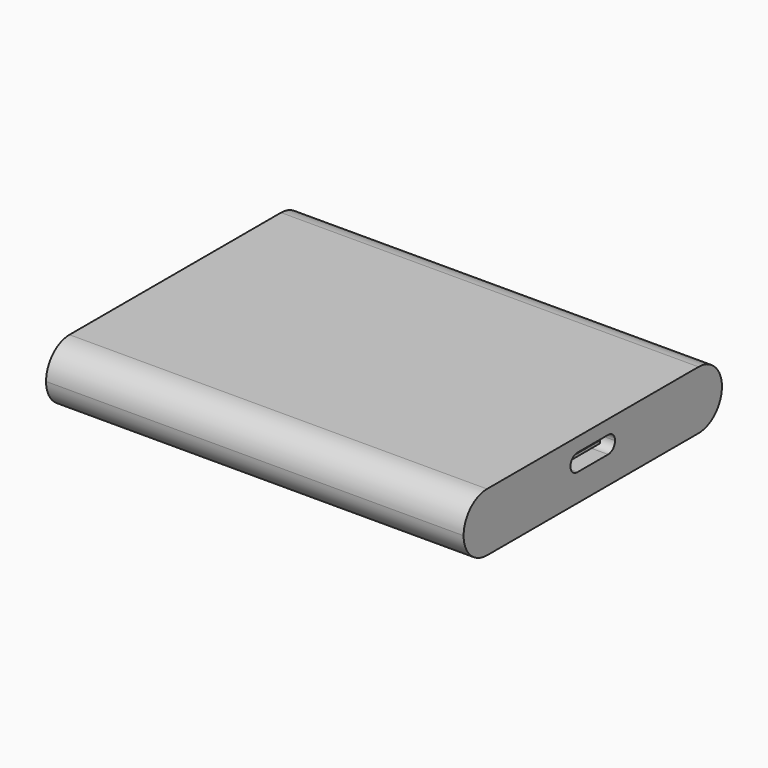
from build123d import *

# Parameters (mm, degrees)
F0_W     = 75
F0_H     = 58
F1_DEPTH = 10.5
F3_R     = 5.24999
F4_DEPTH = 6
F5_W     = 6.9
F5_H     = 0.25
F6_DEPTH = 4.572


# Not quite as in the source:
# - a fillet or chamfer is up to 0.001 mm smaller than in the source, because OpenCascade refuses the exact size


with BuildPart() as f1:
    # F0 (on Top) → F1 (new body)
    with BuildSketch(Plane.XY):
        with Locations((-17.9516240954, -13.4977242947)):
            Rectangle(F0_W, F0_H)
    extrude(amount=F1_DEPTH)

    # F3 (radius 5.25 in the source; OpenCascade refuses exactly that, so slightly less here)
    f3_edges = [f1.edges().sort_by_distance(p)[0] for p in [
        (-17.951624, -42.497724, 10.5),
        (-17.951624, -42.497724, 0),
        (-17.951624, 15.502276, 10.5),
        (-17.951624, 15.502276, 0),
    ]]
    fillet(f3_edges, radius=F3_R)

    # F2 (on face) → F4 (cut)
    with BuildSketch(Plane.YZ.offset(19.5483759046)):
        with BuildLine():
            Line((-10.0477242947, 8), (-13.4977242947, 8))
            Line((-13.4977242947, 8), (-16.9477242947, 8))
            ThreePointArc((-16.9477242947, 8), (-15.8517087838, 7.5460155108), (-15.3977242947, 6.45))
            ThreePointArc((-15.3977242947, 6.45), (-15.8517087838, 5.3539844892), (-16.9477242947, 4.9))
            Line((-16.9477242947, 4.9), (-10.0477242947, 4.9))
            ThreePointArc((-10.0477242947, 4.9), (-11.5977242947, 6.45), (-10.0477242947, 8))
        make_face()
        with BuildLine():
            Line((-10.0477242947, 4.9), (-10.0477242947, 8))
            ThreePointArc((-10.0477242947, 8), (-11.5977242947, 6.45), (-10.0477242947, 4.9))
        make_face()
        with BuildLine():
            ThreePointArc((-8.4977242947, 6.45), (-8.9517087838, 7.5460155108), (-10.0477242947, 8))
            Line((-10.0477242947, 8), (-10.0477242947, 4.9))
            ThreePointArc((-10.0477242947, 4.9), (-8.9517087838, 5.3539844892), (-8.4977242947, 6.45))
        make_face()
        with BuildLine():
            ThreePointArc((-15.3977242947, 6.45), (-15.8517087838, 7.5460155108), (-16.9477242947, 8))
            Line((-16.9477242947, 8), (-16.9477242947, 4.9))
            ThreePointArc((-16.9477242947, 4.9), (-15.8517087838, 5.3539844892), (-15.3977242947, 6.45))
        make_face()
        with BuildLine():
            Line((-16.9477242947, 4.9), (-16.9477242947, 8))
            ThreePointArc((-16.9477242947, 8), (-18.0437398055, 7.5460155108), (-18.4977242947, 6.45))
            ThreePointArc((-18.4977242947, 6.45), (-18.0437398055, 5.3539844892), (-16.9477242947, 4.9))
        make_face()
    extrude(amount=-F4_DEPTH, mode=Mode.SUBTRACT)

    # F5 (on face) → F6 (join)
    with BuildSketch(Plane.YZ.offset(13.5483759046)):
        with Locations((-13.4977242947, 6.575)):
            Rectangle(F5_W, F5_H)
        with Locations((-13.4977242947, 6.325)):
            Rectangle(F5_W, F5_H)
    extrude(amount=F6_DEPTH)


solid = f1.part
